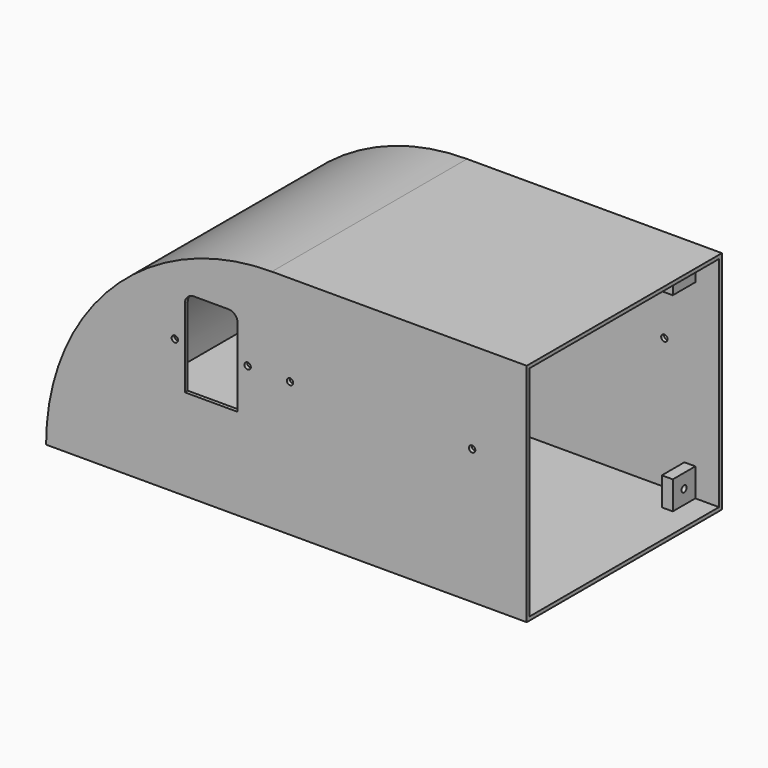
from build123d import *

# Parameters (mm, degrees)
F0_W      = 264
F0_H      = 134
F1_DEPTH  = 62
F3_DEPTH  = 150
F7_START  = -33.8
F7_DEPTH  = 66.4
F8_T      = -2
F9_R      = 1.75
F10_DEPTH = 134.001
F11_R     = 1.75
F12_DEPTH = 25
F14_START = -13
F13_W     = 15.5
F13_H     = 15.5
F13_R     = 1.75
F14_DEPTH = 6


# Not quite as in the source:
# - a feature of the source that left no trace in its solid (it failed there, or was rolled back) is left out


with BuildPart() as f1:
    # F0 (on Top) → F1 (new body, symmetric)
    with BuildSketch(Plane.XY):
        Rectangle(F0_W, F0_H)
    extrude(amount=F1_DEPTH, both=True)

    # F2 (on face) → F3 (cut)
    with BuildSketch(Plane.XZ.offset(67)):
        with BuildLine():
            ThreePointArc((-132, -62), (-95.6812408671, 25.6812408671), (-8, 62))
            Line((-8, 62), (-132, 62))
            Line((-132, 62), (-132, -62))
        make_face()
    extrude(amount=-F3_DEPTH, mode=Mode.SUBTRACT)

    # F6 (on face) → F7 (cut)
    with BuildSketch(Plane.XZ.offset(67).offset(F7_START)):
        Polygon((-105.1785842524, 21.3899467149), (-98.1075164406, 14.318878903), (-86.8645186197, 25.5618767239), (-93.9355864316, 32.6329445358), align=None)
    extrude(amount=-F7_DEPTH, mode=Mode.SUBTRACT)

    # F8
    f8_openings = [f1.faces().sort_by_distance(p)[0] for p in [
        (132, 0, 0),
    ]]
    offset(amount=F8_T, openings=f8_openings, kind=Kind.INTERSECTION)

    # F9 (on face) → F10 (cut, through all)
    with BuildSketch(Plane.XZ.offset(67)):
        with Locations((102, 12)):
            Circle(F9_R)
        with Locations((2, 12)):
            Circle(F9_R)
    extrude(amount=-F10_DEPTH, mode=Mode.SUBTRACT)

    # F11 (on face) → F12 (cut)
    with BuildSketch(Plane.XZ.offset(67)):
        with BuildLine():
            ThreePointArc((-26.79829216, 31.0818016827), (-28.2627582541, 34.6173355886), (-31.79829216, 36.0818016827))
            Line((-31.79829216, 36.0818016827), (-50.79829216, 36.0818016827))
            ThreePointArc((-50.79829216, 36.0818016827), (-54.333826066, 34.6173355886), (-55.79829216, 31.0818016827))
            Line((-55.79829216, 31.0818016827), (-55.79829216, -11.9181983173))
            Line((-55.79829216, -11.9181983173), (-26.79829216, -11.9181983173))
            Line((-26.79829216, -11.9181983173), (-26.79829216, 31.0818016827))
        make_face()
        with Locations((-61.29829216, 12.0818016827)):
            Circle(F11_R)
        with Locations((-21.29829216, 12.0818016827)):
            Circle(F11_R)
    extrude(amount=-F12_DEPTH, mode=Mode.SUBTRACT)

    # F13 (on face) → F14 (join)
    with BuildSketch(Plane.YZ.offset(132).offset(F14_START)):
        with Locations((-57.25, 52.25)):
            Rectangle(F13_W, F13_H)
        with Locations((-57.25, 52.25)):
            Circle(F13_R, mode=Mode.SUBTRACT)
        with Locations((57.25, 52.25)):
            Rectangle(F13_W, F13_H)
        with Locations((57.25, 52.25)):
            Circle(F13_R, mode=Mode.SUBTRACT)
        with Locations((57.25, -52.25)):
            Rectangle(F13_W, F13_H)
        with Locations((57.25, -52.25)):
            Circle(F13_R, mode=Mode.SUBTRACT)
        with Locations((-57.25, -52.25)):
            Rectangle(F13_W, F13_H)
        with Locations((-57.25, -52.25)):
            Circle(F13_R, mode=Mode.SUBTRACT)
    extrude(amount=-F14_DEPTH)


solid = f1.part
